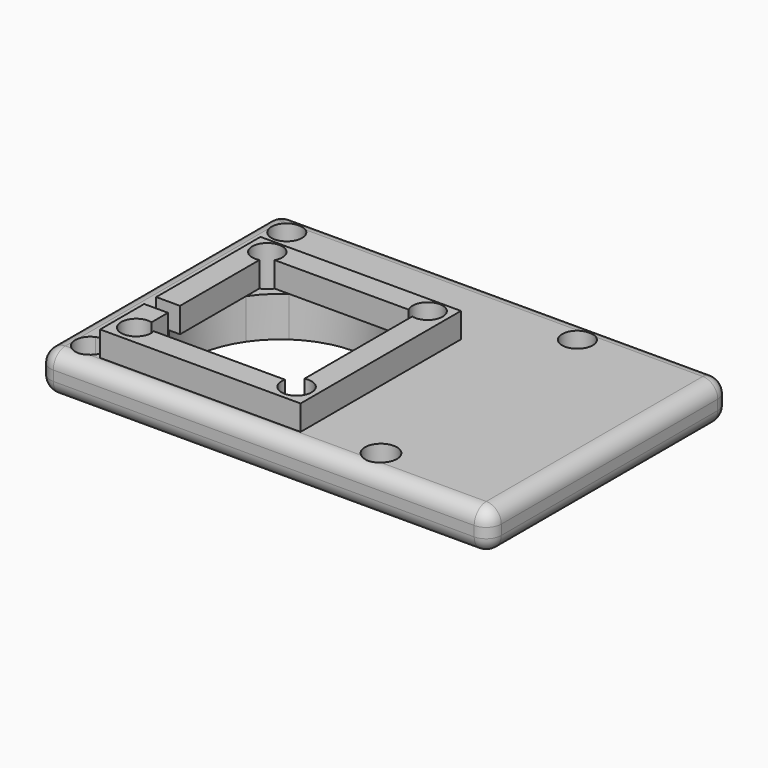
from build123d import *

# Parameters (mm, degrees)
F0_W         = 40
F0_H         = 40
F1_DEPTH     = 5
F0_R         = 3.1797922952
F0_R_2       = 3.05
F0_R_3       = 1.375
F2_DEPTH     = 8
F4_DEPTH     = 10
F5_DEPTH     = 5
F7_DEPTH     = 13.001
F8_T1_DEPTH  = 84
F8_T3_DEPTH  = 54
F8_T6_ANGLE  = 90
F8_T8_ANGLE  = 90
F8_T10_ANGLE = 90
F8_T12_ANGLE = 90
F8_T14_ANGLE = 90
F8_T16_ANGLE = 90
F8_T18_ANGLE = 90
F8_T20_ANGLE = 90


# Not quite as in the source:
# - a fillet or chamfer that OpenCascade refuses, or shapes differently, is made with other operations: its cross-section is extruded or revolved along the edge and cut away or added


with BuildPart() as f1:
    # F0 (on Top) → F1 (new body)
    with BuildSketch(Plane.XY):
        with Locations((-19.0296009332, 0)):
            Rectangle(F0_W, F0_H)
        with BuildLine():
            Line((-29.502780966, -15.25), (-33.5599070875, -15.25))
            ThreePointArc((-33.5599070875, -15.25), (-33.4253106157, -15.6143154432), (-33.3796009332, -16))
            ThreePointArc((-33.3796009332, -16), (-36.4367256611, -16.861684397), (-34.2796009332, -14.5303061543))
            Line((-34.2796009332, -14.5303061543), (-34.2796009332, -10.4731800328))
            ThreePointArc((-34.2796009332, -10.4731800328), (-37.5296009332, 0), (-34.2796009332, 10.4731800328))
            Line((-34.2796009332, 10.4731800328), (-34.2796009332, 15.2303061543))
            ThreePointArc((-34.2796009332, 15.2303061543), (-36.4367256611, 17.561684397), (-33.3796009332, 16.7))
            ThreePointArc((-33.3796009332, 16.7), (-33.6115545131, 15.8564098445), (-34.2422001458, 15.25))
            Line((-34.2422001458, 15.25), (-29.502780966, 15.25))
            ThreePointArc((-29.502780966, 15.25), (-19.0296009332, 18.5), (-8.5564209004, 15.25))
            Line((-8.5564209004, 15.25), (-3.8170017206, 15.25))
            ThreePointArc((-3.8170017206, 15.25), (-3.8731910887, 18.1180464201), (-1.3796009332, 16.7))
            ThreePointArc((-1.3796009332, 16.7), (-2.1679165362, 15.2928752721), (-3.7796009332, 15.2303061543))
            Line((-3.7796009332, 15.2303061543), (-3.7796009332, 10.4731800328))
            ThreePointArc((-3.7796009332, 10.4731800328), (-1.3607724491, 5.4829280499), (-0.5296009332, 0))
            ThreePointArc((-0.5296009332, 0), (-1.3607724491, -5.4829280499), (-3.7796009332, -10.4731800328))
            Line((-3.7796009332, -10.4731800328), (-3.7796009332, -14.5303061543))
            ThreePointArc((-3.7796009332, -14.5303061543), (-2.1679165362, -14.5928752721), (-1.3796009332, -16))
            ThreePointArc((-1.3796009332, -16), (-3.41528549, -17.6042903175), (-4.4992947789, -15.25))
            Line((-4.4992947789, -15.25), (-8.5564209004, -15.25))
            ThreePointArc((-8.5564209004, -15.25), (-19.0296009332, -18.5), (-29.502780966, -15.25))
        make_face(mode=Mode.SUBTRACT)
        with BuildLine():
            Line((-8.5564209004, -15.25), (-29.502780966, -15.25))
            ThreePointArc((-29.502780966, -15.25), (-19.0296009332, -18.5), (-8.5564209004, -15.25))
        make_face()
        with BuildLine():
            Line((-3.7796009332, 10.4731800328), (-3.7796009332, -10.4731800328))
            ThreePointArc((-3.7796009332, -10.4731800328), (-1.3607724491, -5.4829280499), (-0.5296009332, 0))
            ThreePointArc((-0.5296009332, 0), (-1.3607724491, 5.4829280499), (-3.7796009332, 10.4731800328))
        make_face()
        with BuildLine():
            ThreePointArc((-8.5564209004, 15.25), (-19.0296009332, 18.5), (-29.502780966, 15.25))
            Line((-29.502780966, 15.25), (-8.5564209004, 15.25))
        make_face()
        with BuildLine():
            ThreePointArc((-34.2796009332, 10.4731800328), (-37.5296009332, 0), (-34.2796009332, -10.4731800328))
            Line((-34.2796009332, -10.4731800328), (-34.2796009332, 10.4731800328))
        make_face()
    extrude(amount=F1_DEPTH)

    # F0 (on Top) → F2 (join)
    with BuildSketch(Plane.XY):
        with BuildLine():
            ThreePointArc((-48.7796009332, -20.25), (-47.9009212768, -22.3713203436), (-45.7796009332, -23.25))
            Line((-45.7796009332, -23.25), (38.2203990668, -23.25))
            ThreePointArc((38.2203990668, -23.25), (40.3417194104, -22.3713203436), (41.2203990668, -20.25))
            Line((41.2203990668, -20.25), (41.2203990668, 33.75))
            ThreePointArc((41.2203990668, 33.75), (40.3417194104, 35.8713203436), (38.2203990668, 36.75))
            Line((38.2203990668, 36.75), (-45.7796009332, 36.75))
            ThreePointArc((-45.7796009332, 36.75), (-47.9009212768, 35.8713203436), (-48.7796009332, 33.75))
            Line((-48.7796009332, 33.75), (-48.7796009332, -20.25))
        make_face()
        with BuildLine():
            ThreePointArc((-41.0324604122, -20.25), (-45.4323154128, -19.2551929743), (-44.0296009332, -14.9679144514))
            Line((-44.0296009332, -14.9679144514), (-44.0296009332, 24.75))
            Line((-44.0296009332, 24.75), (5.9703990668, 24.75))
            Line((5.9703990668, 24.75), (5.9703990668, -20.25))
            Line((5.9703990668, -20.25), (-41.0324604122, -20.25))
        make_face(mode=Mode.SUBTRACT)
        with Locations((15.2203990668, -17.75)):
            Circle(F0_R, mode=Mode.SUBTRACT)
        with Locations((-42.7796009332, 31.25)):
            Circle(F0_R_2, mode=Mode.SUBTRACT)
        with Locations((15.2203990668, 31.25)):
            Circle(F0_R_2, mode=Mode.SUBTRACT)
        with BuildLine():
            Line((-44.0296009332, 24.75), (-44.0296009332, -14.9679144514))
            ThreePointArc((-44.0296009332, -14.9679144514), (-41.1227967806, -15.1892383945), (-39.7296009332, -17.75))
            ThreePointArc((-39.7296009332, -17.75), (-40.0748570831, -19.1595604654), (-41.0324604122, -20.25))
            Line((-41.0324604122, -20.25), (5.9703990668, -20.25))
            Line((5.9703990668, -20.25), (5.9703990668, 24.75))
            Line((5.9703990668, 24.75), (-44.0296009332, 24.75))
        make_face()
        with Locations((-19.0296009332, 0)):
            Rectangle(F0_W, F0_H, mode=Mode.SUBTRACT)
        with Locations((-19.0296009332, 0)):
            Rectangle(F0_W, F0_H)
        with BuildLine():
            Line((-29.502780966, -15.25), (-33.5599070875, -15.25))
            ThreePointArc((-33.5599070875, -15.25), (-33.4253106157, -15.6143154432), (-33.3796009332, -16))
            ThreePointArc((-33.3796009332, -16), (-36.4367256611, -16.861684397), (-34.2796009332, -14.5303061543))
            Line((-34.2796009332, -14.5303061543), (-34.2796009332, -10.4731800328))
            ThreePointArc((-34.2796009332, -10.4731800328), (-37.5296009332, 0), (-34.2796009332, 10.4731800328))
            Line((-34.2796009332, 10.4731800328), (-34.2796009332, 15.2303061543))
            ThreePointArc((-34.2796009332, 15.2303061543), (-36.4367256611, 17.561684397), (-33.3796009332, 16.7))
            ThreePointArc((-33.3796009332, 16.7), (-33.6115545131, 15.8564098445), (-34.2422001458, 15.25))
            Line((-34.2422001458, 15.25), (-29.502780966, 15.25))
            ThreePointArc((-29.502780966, 15.25), (-19.0296009332, 18.5), (-8.5564209004, 15.25))
            Line((-8.5564209004, 15.25), (-3.8170017206, 15.25))
            ThreePointArc((-3.8170017206, 15.25), (-3.8731910887, 18.1180464201), (-1.3796009332, 16.7))
            ThreePointArc((-1.3796009332, 16.7), (-2.1679165362, 15.2928752721), (-3.7796009332, 15.2303061543))
            Line((-3.7796009332, 15.2303061543), (-3.7796009332, 10.4731800328))
            ThreePointArc((-3.7796009332, 10.4731800328), (-1.3607724491, 5.4829280499), (-0.5296009332, 0))
            ThreePointArc((-0.5296009332, 0), (-1.3607724491, -5.4829280499), (-3.7796009332, -10.4731800328))
            Line((-3.7796009332, -10.4731800328), (-3.7796009332, -14.5303061543))
            ThreePointArc((-3.7796009332, -14.5303061543), (-2.1679165362, -14.5928752721), (-1.3796009332, -16))
            ThreePointArc((-1.3796009332, -16), (-3.41528549, -17.6042903175), (-4.4992947789, -15.25))
            Line((-4.4992947789, -15.25), (-8.5564209004, -15.25))
            ThreePointArc((-8.5564209004, -15.25), (-19.0296009332, -18.5), (-29.502780966, -15.25))
        make_face(mode=Mode.SUBTRACT)
        with Locations((15.2203990668, -17.75)):
            Circle(F0_R)
        with Locations((15.2203990668, -17.75)):
            Circle(F0_R_3, mode=Mode.SUBTRACT)
        with Locations((15.2203990668, 31.25)):
            Circle(F0_R_2)
        with Locations((15.2203990668, 31.25)):
            Circle(F0_R_3, mode=Mode.SUBTRACT)
        with Locations((-42.7796009332, 31.25)):
            Circle(F0_R_2)
        with Locations((-42.7796009332, 31.25)):
            Circle(F0_R_3, mode=Mode.SUBTRACT)
        with BuildLine():
            ThreePointArc((-44.0296009332, -17.1771780381), (-42.4864499482, -16.4066134212), (-41.4046009332, -17.75))
            ThreePointArc((-41.4046009332, -17.75), (-42.4864499482, -19.0933865788), (-44.0296009332, -18.3228219619))
            Line((-44.0296009332, -18.3228219619), (-44.0296009332, -20.25))
            Line((-44.0296009332, -20.25), (-41.0324604122, -20.25))
            ThreePointArc((-41.0324604122, -20.25), (-40.0748570831, -19.1595604654), (-39.7296009332, -17.75))
            ThreePointArc((-39.7296009332, -17.75), (-41.1227967806, -15.1892383945), (-44.0296009332, -14.9679144514))
            Line((-44.0296009332, -14.9679144514), (-44.0296009332, -17.1771780381))
        make_face()
        with BuildLine():
            ThreePointArc((-8.5564209004, 15.25), (-5.9481254812, 13.081475452), (-3.7796009332, 10.4731800328))
            Line((-3.7796009332, 10.4731800328), (-3.7796009332, 15.2303061543))
            ThreePointArc((-3.7796009332, 15.2303061543), (-3.798364393, 15.2400333076), (-3.8170017206, 15.25))
            Line((-3.8170017206, 15.25), (-8.5564209004, 15.25))
        make_face()
        with BuildLine():
            Line((-34.2796009332, 15.2303061543), (-34.2796009332, 10.4731800328))
            ThreePointArc((-34.2796009332, 10.4731800328), (-32.1110763851, 13.081475452), (-29.502780966, 15.25))
            Line((-29.502780966, 15.25), (-34.2422001458, 15.25))
            ThreePointArc((-34.2422001458, 15.25), (-34.2608374734, 15.2400333076), (-34.2796009332, 15.2303061543))
        make_face()
        with BuildLine():
            ThreePointArc((-3.7796009332, -10.4731800328), (-5.9481254812, -13.081475452), (-8.5564209004, -15.25))
            Line((-8.5564209004, -15.25), (-4.4992947789, -15.25))
            ThreePointArc((-4.4992947789, -15.25), (-4.1963271222, -14.833273811), (-3.7796009332, -14.5303061543))
            Line((-3.7796009332, -14.5303061543), (-3.7796009332, -10.4731800328))
        make_face()
        with BuildLine():
            ThreePointArc((-34.2796009332, -14.5303061543), (-33.8628747442, -14.833273811), (-33.5599070875, -15.25))
            Line((-33.5599070875, -15.25), (-29.502780966, -15.25))
            ThreePointArc((-29.502780966, -15.25), (-32.1110763851, -13.081475452), (-34.2796009332, -10.4731800328))
            Line((-34.2796009332, -10.4731800328), (-34.2796009332, -14.5303061543))
        make_face()
        with BuildLine():
            ThreePointArc((-44.0296009332, -18.3228219619), (-44.1546009332, -17.75), (-44.0296009332, -17.1771780381))
            Line((-44.0296009332, -17.1771780381), (-44.0296009332, -14.9679144514))
            ThreePointArc((-44.0296009332, -14.9679144514), (-45.4323154128, -19.2551929743), (-41.0324604122, -20.25))
            Line((-41.0324604122, -20.25), (-44.0296009332, -20.25))
            Line((-44.0296009332, -20.25), (-44.0296009332, -18.3228219619))
        make_face()
        with BuildLine():
            ThreePointArc((-3.8170017206, 15.25), (-3.798364393, 15.2400333076), (-3.7796009332, 15.2303061543))
            Line((-3.7796009332, 15.2303061543), (-3.7796009332, 15.25))
            Line((-3.7796009332, 15.25), (-3.8170017206, 15.25))
        make_face()
        with BuildLine():
            Line((-34.2796009332, 15.25), (-34.2796009332, 15.2303061543))
            ThreePointArc((-34.2796009332, 15.2303061543), (-34.2608374734, 15.2400333076), (-34.2422001458, 15.25))
            Line((-34.2422001458, 15.25), (-34.2796009332, 15.25))
        make_face()
    extrude(amount=-F2_DEPTH)

    # F3 (on face) → F4 (cut)
    with BuildSketch(Plane.XY.offset(5)):
        with BuildLine():
            Line((-34.2796009332, 15.2303061543), (-34.2796009332, 13.7952624903))
            ThreePointArc((-34.2796009332, 13.7952624903), (-33.1914139855, 14.3291206809), (-32.4032917359, 15.25))
            Line((-32.4032917359, 15.25), (-34.2422001458, 15.25))
            ThreePointArc((-34.2422001458, 15.25), (-35.798364393, 18.1599666924), (-34.2796009332, 15.2303061543))
        make_face()
        with BuildLine():
            ThreePointArc((-32.1248634235, -15.25), (-32.9082805896, -13.8786796564), (-34.2796009332, -13.0952624903))
            Line((-34.2796009332, -13.0952624903), (-34.2796009332, -14.5303061543))
            ThreePointArc((-34.2796009332, -14.5303061543), (-36.1963271222, -17.166726189), (-33.5599070875, -15.25))
            Line((-33.5599070875, -15.25), (-32.1248634235, -15.25))
        make_face()
        with BuildLine():
            ThreePointArc((-32.4032917359, 15.25), (-32.1245254099, 15.951310342), (-32.0296009332, 16.7))
            ThreePointArc((-32.0296009332, 16.7), (-37.4013091783, 18.5371173071), (-34.2796009332, 13.7952624903))
            Line((-34.2796009332, 13.7952624903), (-34.2796009332, 15.2303061543))
            ThreePointArc((-34.2796009332, 15.2303061543), (-35.798364393, 18.1599666924), (-34.2422001458, 15.25))
            Line((-34.2422001458, 15.25), (-32.4032917359, 15.25))
        make_face()
        with BuildLine():
            Line((-34.2796009332, -14.5303061543), (-34.2796009332, -13.0952624903))
            ThreePointArc((-34.2796009332, -13.0952624903), (-37.4013091783, -17.8371173071), (-32.0296009332, -16))
            ThreePointArc((-32.0296009332, -16), (-32.0535118444, -15.6219871226), (-32.1248634235, -15.25))
            Line((-32.1248634235, -15.25), (-33.5599070875, -15.25))
            ThreePointArc((-33.5599070875, -15.25), (-36.1963271222, -17.166726189), (-34.2796009332, -14.5303061543))
        make_face()
        with BuildLine():
            ThreePointArc((-3.7796009332, -13.0952624903), (-5.1509212768, -13.8786796564), (-5.9343384428, -15.25))
            Line((-5.9343384428, -15.25), (-4.4992947789, -15.25))
            ThreePointArc((-4.4992947789, -15.25), (-1.8628747442, -17.166726189), (-3.7796009332, -14.5303061543))
            Line((-3.7796009332, -14.5303061543), (-3.7796009332, -13.0952624903))
        make_face()
        with BuildLine():
            Line((-4.4992947789, -15.25), (-5.9343384428, -15.25))
            ThreePointArc((-5.9343384428, -15.25), (-3.4076138106, -18.9760890888), (-0.0296009332, -16))
            ThreePointArc((-0.0296009332, -16), (-1.1924836261, -13.6282917549), (-3.7796009332, -13.0952624903))
            Line((-3.7796009332, -13.0952624903), (-3.7796009332, -14.5303061543))
            ThreePointArc((-3.7796009332, -14.5303061543), (-1.8628747442, -17.166726189), (-4.4992947789, -15.25))
        make_face()
        with BuildLine():
            Line((-3.8170017206, 15.25), (-5.6559101305, 15.25))
            ThreePointArc((-5.6559101305, 15.25), (-4.8677878808, 14.3291206809), (-3.7796009332, 13.7952624903))
            Line((-3.7796009332, 13.7952624903), (-3.7796009332, 15.2303061543))
            ThreePointArc((-3.7796009332, 15.2303061543), (-2.2608374734, 18.1599666924), (-3.8170017206, 15.25))
        make_face()
        with BuildLine():
            ThreePointArc((-0.0296009332, 16.7), (-3.7782905912, 19.6050755233), (-5.6559101305, 15.25))
            Line((-5.6559101305, 15.25), (-3.8170017206, 15.25))
            ThreePointArc((-3.8170017206, 15.25), (-2.2608374734, 18.1599666924), (-3.7796009332, 15.2303061543))
            Line((-3.7796009332, 15.2303061543), (-3.7796009332, 13.7952624903))
            ThreePointArc((-3.7796009332, 13.7952624903), (-1.1924836261, 14.3282917549), (-0.0296009332, 16.7))
        make_face()
    extrude(amount=-F4_DEPTH, mode=Mode.SUBTRACT)

    # F0 (on Top) → F5 (cut)
    with BuildSketch(Plane.XY):
        with BuildLine():
            ThreePointArc((-44.0296009332, -18.3228219619), (-44.1546009332, -17.75), (-44.0296009332, -17.1771780381))
            Line((-44.0296009332, -17.1771780381), (-44.0296009332, -14.9679144514))
            ThreePointArc((-44.0296009332, -14.9679144514), (-45.4323154128, -19.2551929743), (-41.0324604122, -20.25))
            Line((-41.0324604122, -20.25), (-44.0296009332, -20.25))
            Line((-44.0296009332, -20.25), (-44.0296009332, -18.3228219619))
        make_face()
        with BuildLine():
            ThreePointArc((-44.0296009332, -17.1771780381), (-42.4864499482, -16.4066134212), (-41.4046009332, -17.75))
            ThreePointArc((-41.4046009332, -17.75), (-42.4864499482, -19.0933865788), (-44.0296009332, -18.3228219619))
            Line((-44.0296009332, -18.3228219619), (-44.0296009332, -20.25))
            Line((-44.0296009332, -20.25), (-41.0324604122, -20.25))
            ThreePointArc((-41.0324604122, -20.25), (-40.0748570831, -19.1595604654), (-39.7296009332, -17.75))
            ThreePointArc((-39.7296009332, -17.75), (-41.1227967806, -15.1892383945), (-44.0296009332, -14.9679144514))
            Line((-44.0296009332, -14.9679144514), (-44.0296009332, -17.1771780381))
        make_face()
        with Locations((15.2203990668, -17.75)):
            Circle(F0_R)
        with Locations((15.2203990668, -17.75)):
            Circle(F0_R_3, mode=Mode.SUBTRACT)
        with Locations((15.2203990668, 31.25)):
            Circle(F0_R_2)
        with Locations((15.2203990668, 31.25)):
            Circle(F0_R_3, mode=Mode.SUBTRACT)
        with Locations((-42.7796009332, 31.25)):
            Circle(F0_R_2)
        with Locations((-42.7796009332, 31.25)):
            Circle(F0_R_3, mode=Mode.SUBTRACT)
    extrude(amount=-F5_DEPTH, mode=Mode.SUBTRACT)

    # F6 (on face) → F7 (cut, through all)
    with BuildSketch(Plane(origin=(0, 0, -8), x_dir=(1, 0, 0), z_dir=(0, 0, -1))):
        with BuildLine():
            ThreePointArc((-38.9575995505, 6.0132511556), (-37.8969393787, 6.4525909838), (-37.4575995505, 7.5132511556))
            ThreePointArc((-37.4575995505, 7.5132511556), (-37.8969393787, 8.5739113274), (-38.9575995505, 9.0132511556))
            ThreePointArc((-38.9575995505, 9.0132511556), (-40.4575995505, 7.5132511556), (-38.9575995505, 6.0132511556))
        make_face()
        with BuildLine():
            ThreePointArc((-38.9575995505, 9.0132511556), (-37.8969393787, 8.5739113274), (-37.4575995505, 7.5132511556))
            ThreePointArc((-37.4575995505, 7.5132511556), (-37.8969393787, 6.4525909838), (-38.9575995505, 6.0132511556))
            Line((-38.9575995505, 6.0132511556), (-36.5250520717, 6.0132511556))
            ThreePointArc((-36.5250520717, 6.0132511556), (-35.9219785167, 7.5430484274), (-35.1854451886, 9.0132511556))
            Line((-35.1854451886, 9.0132511556), (-38.9575995505, 9.0132511556))
        make_face()
        with BuildLine():
            Line((-34.0454205871, 9.0132511556), (-35.1854451886, 9.0132511556))
            ThreePointArc((-35.1854451886, 9.0132511556), (-35.9219785167, 7.5430484274), (-36.5250520717, 6.0132511556))
            Line((-36.5250520717, 6.0132511556), (-34.0454205871, 6.0132511556))
            Line((-34.0454205871, 6.0132511556), (-34.0454205871, 9.0132511556))
        make_face()
    extrude(amount=-F7_DEPTH, mode=Mode.SUBTRACT)

    # F8: fillet of radius 3 on 16 edges, made by hand

    # F8_s2 → F8_t1 (cut)
    with BuildSketch(Plane.YZ.offset(-45.7796009332)):
        with BuildLine():
            ThreePointArc((-20.25, 0), (-22.3713203436, -0.8786796564), (-23.25, -3))
            Line((-23.25, -3), (-23.25, 0))
            Line((-23.25, 0), (-20.25, 0))
        make_face()
        with BuildLine():
            ThreePointArc((-20.25, -8), (-22.3713203436, -7.1213203436), (-23.25, -5))
            Line((-23.25, -5), (-23.25, -8))
            Line((-23.25, -8), (-20.25, -8))
        make_face()
        with BuildLine():
            ThreePointArc((33.75, -8), (35.8713203436, -7.1213203436), (36.75, -5))
            Line((36.75, -5), (36.75, -8))
            Line((36.75, -8), (33.75, -8))
        make_face()
        with BuildLine():
            ThreePointArc((33.75, 0), (35.8713203436, -0.8786796564), (36.75, -3))
            Line((36.75, -3), (36.75, 0))
            Line((36.75, 0), (33.75, 0))
        make_face()
    extrude(amount=F8_T1_DEPTH, mode=Mode.SUBTRACT)

    # F8_s4 → F8_t3 (cut)
    with BuildSketch(Plane.XZ.offset(-33.75)):
        with BuildLine():
            ThreePointArc((-45.7796009332, -8), (-47.9009212768, -7.1213203436), (-48.7796009332, -5))
            Line((-48.7796009332, -5), (-48.7796009332, -8))
            Line((-48.7796009332, -8), (-45.7796009332, -8))
        make_face()
        with BuildLine():
            ThreePointArc((38.2203990668, -8), (40.3417194104, -7.1213203436), (41.2203990668, -5))
            Line((41.2203990668, -5), (41.2203990668, -8))
            Line((41.2203990668, -8), (38.2203990668, -8))
        make_face()
        with BuildLine():
            ThreePointArc((-45.7796009332, 0), (-47.9009212768, -0.8786796564), (-48.7796009332, -3))
            Line((-48.7796009332, -3), (-48.7796009332, 0))
            Line((-48.7796009332, 0), (-45.7796009332, 0))
        make_face()
        with BuildLine():
            ThreePointArc((38.2203990668, 0), (40.3417194104, -0.8786796564), (41.2203990668, -3))
            Line((41.2203990668, -3), (41.2203990668, 0))
            Line((41.2203990668, 0), (38.2203990668, 0))
        make_face()
    extrude(amount=F8_T3_DEPTH, mode=Mode.SUBTRACT)

    # F8_s5 → F8_t6 (revolve, cut)
    with BuildSketch(Plane.YZ.offset(-45.7796009332)):
        with BuildLine():
            ThreePointArc((33.75, -8), (35.8713203436, -7.1213203436), (36.75, -5))
            Line((36.75, -5), (36.75, -8))
            Line((36.75, -8), (33.75, -8))
        make_face()
    revolve(axis=Axis((-45.7796009332, 33.75, -8), (0, 0, 1)), revolution_arc=F8_T6_ANGLE, mode=Mode.SUBTRACT)

    # F8_s7 → F8_t8 (revolve, cut)
    with BuildSketch(Plane.XZ.offset(20.25)):
        with BuildLine():
            ThreePointArc((-45.7796009332, -8), (-47.9009212768, -7.1213203436), (-48.7796009332, -5))
            Line((-48.7796009332, -5), (-48.7796009332, -8))
            Line((-48.7796009332, -8), (-45.7796009332, -8))
        make_face()
    revolve(axis=Axis((-45.7796009332, -20.25, -8), (0, 0, 1)), revolution_arc=F8_T8_ANGLE, mode=Mode.SUBTRACT)

    # F8_s9 → F8_t10 (revolve, cut)
    with BuildSketch(Plane.YZ.offset(38.2203990668)):
        with BuildLine():
            ThreePointArc((-20.25, -8), (-22.3713203436, -7.1213203436), (-23.25, -5))
            Line((-23.25, -5), (-23.25, -8))
            Line((-23.25, -8), (-20.25, -8))
        make_face()
    revolve(axis=Axis((38.2203990668, -20.25, -8), (0, 0, 1)), revolution_arc=F8_T10_ANGLE, mode=Mode.SUBTRACT)

    # F8_s11 → F8_t12 (revolve, cut)
    with BuildSketch(Plane.XZ.offset(-33.75)):
        with BuildLine():
            ThreePointArc((38.2203990668, -8), (40.3417194104, -7.1213203436), (41.2203990668, -5))
            Line((41.2203990668, -5), (41.2203990668, -8))
            Line((41.2203990668, -8), (38.2203990668, -8))
        make_face()
    revolve(axis=Axis((38.2203990668, 33.75, -8), (0, 0, 1)), revolution_arc=F8_T12_ANGLE, mode=Mode.SUBTRACT)

    # F8_s13 → F8_t14 (revolve, cut)
    with BuildSketch(Plane.YZ.offset(-45.7796009332)):
        with BuildLine():
            ThreePointArc((33.75, 0), (35.8713203436, -0.8786796564), (36.75, -3))
            Line((36.75, -3), (36.75, 0))
            Line((36.75, 0), (33.75, 0))
        make_face()
    revolve(axis=Axis((-45.7796009332, 33.75, 0), (0, 0, 1)), revolution_arc=F8_T14_ANGLE, mode=Mode.SUBTRACT)

    # F8_s15 → F8_t16 (revolve, cut)
    with BuildSketch(Plane.XZ.offset(-33.75)):
        with BuildLine():
            ThreePointArc((38.2203990668, 0), (40.3417194104, -0.8786796564), (41.2203990668, -3))
            Line((41.2203990668, -3), (41.2203990668, 0))
            Line((41.2203990668, 0), (38.2203990668, 0))
        make_face()
    revolve(axis=Axis((38.2203990668, 33.75, 0), (0, 0, 1)), revolution_arc=F8_T16_ANGLE, mode=Mode.SUBTRACT)

    # F8_s17 → F8_t18 (revolve, cut)
    with BuildSketch(Plane.XZ.offset(20.25)):
        with BuildLine():
            ThreePointArc((-45.7796009332, 0), (-47.9009212768, -0.8786796564), (-48.7796009332, -3))
            Line((-48.7796009332, -3), (-48.7796009332, 0))
            Line((-48.7796009332, 0), (-45.7796009332, 0))
        make_face()
    revolve(axis=Axis((-45.7796009332, -20.25, 0), (0, 0, 1)), revolution_arc=F8_T18_ANGLE, mode=Mode.SUBTRACT)

    # F8_s19 → F8_t20 (revolve, cut)
    with BuildSketch(Plane.YZ.offset(38.2203990668)):
        with BuildLine():
            ThreePointArc((-20.25, 0), (-22.3713203436, -0.8786796564), (-23.25, -3))
            Line((-23.25, -3), (-23.25, 0))
            Line((-23.25, 0), (-20.25, 0))
        make_face()
    revolve(axis=Axis((38.2203990668, -20.25, 0), (0, 0, 1)), revolution_arc=F8_T20_ANGLE, mode=Mode.SUBTRACT)


solid = f1.part
